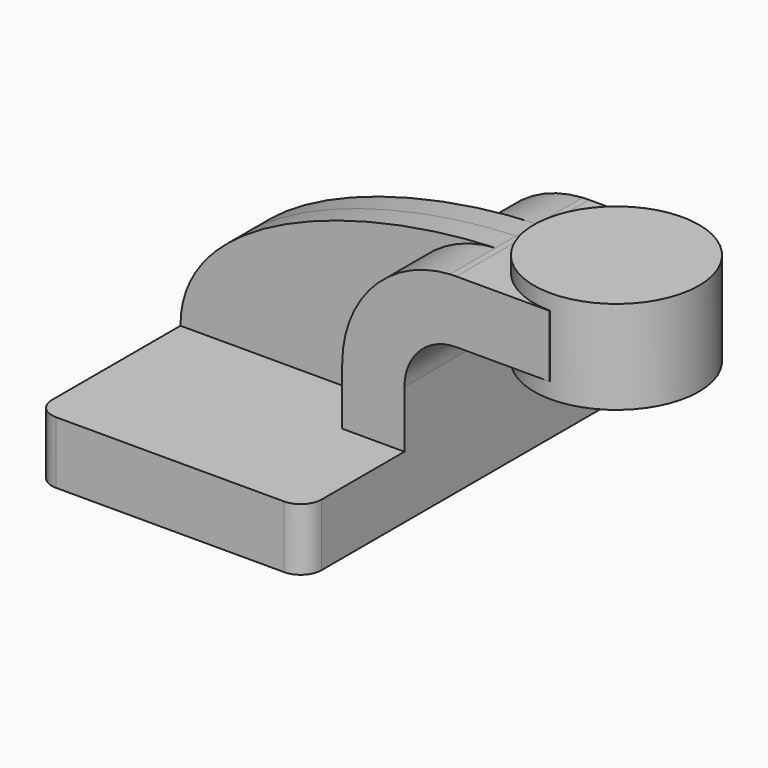
from build123d import *

# Parameters (mm, degrees)
F1_DEPTH = 63.5
F0_W     = 25.4
F0_H     = 19.05
F2_DEPTH = 25.4
F3_DEPTH = 7.9375
F6_R     = 6.35


with BuildPart() as f1:
    # F0 (on Front) → F1 (new body, symmetric)
    with BuildSketch(Plane.XZ):
        Polygon((-41.275, -9.525), (41.275, -9.525), (41.275, 9.525), (22.225, 9.525), (-41.275, 9.525), align=None)
    extrude(amount=F1_DEPTH, both=True)

    # F0 (on Front) → F2 (join, symmetric)
    with BuildSketch(Plane.XZ):
        with BuildLine():
            Line((22.225, 9.525), (41.275, 9.525))
            Line((41.275, 9.525), (41.275, 27.0002))
            ThreePointArc((41.275, 27.0002), (45.9246798487, 38.2255201513), (57.15, 42.8752))
            Line((57.15, 42.8752), (60.325, 42.8752))
            Line((60.325, 42.8752), (60.325, 61.9252))
            Line((60.325, 61.9252), (57.15, 61.9252))
            add(Edge.make_bspline(
                [(55.1794589503, 61.8695646769), (55.8399698658, 61.8922829135), (56.4969113909, 61.9108291292), (57.15, 61.9252)],
                knots=[109.7486555894, 109.7486555894, 109.7486555894, 109.7486555894, 111.5045361635, 111.5045361635, 111.5045361635, 111.5045361635], degree=3))
            ThreePointArc((55.1794589503, 61.8695646769), (31.7671635631, 50.9890982536), (22.225, 27.0002))
            Line((22.225, 27.0002), (22.225, 9.525))
        make_face()
        with Locations((73.025, 52.4002)):
            Rectangle(F0_W, F0_H)
    extrude(amount=F2_DEPTH, both=True)

    # F0 (on Front) → F3 (join, symmetric)
    with BuildSketch(Plane.XZ):
        with BuildLine():
            add(Edge.make_bspline(
                [(-41.275, 9.525), (-41.3334957388, 42.730852595), (13.8952246787, 60.4495957119), (55.1794589503, 61.8695646769)],
                knots=[0, 0, 0, 0, 109.7486555894, 109.7486555894, 109.7486555894, 109.7486555894], degree=3))
            Line((-41.275, 9.525), (22.225, 9.525))
            Line((22.225, 9.525), (22.225, 27.0002))
            ThreePointArc((22.225, 27.0002), (31.7671635631, 50.9890982536), (55.1794589503, 61.8695646769))
        make_face()
    extrude(amount=F3_DEPTH, both=True)

    # F6
    f6_edges = [f1.edges().sort_by_distance(p)[0] for p in [
        (41.275, 63.5, 0),
        (41.275, -63.5, 0),
        (-41.275, 63.5, 0),
        (-41.275, -63.5, 0),
    ]]
    fillet(f6_edges, radius=F6_R)


with BuildPart() as f5:
    # F4 (on face) → F5 (revolve)
    with BuildSketch(Plane.XZ):
        Polygon((85.8692377806, 66.675), (85.8692377806, 43.0761948228), (85.8692377806, 38.1), (111.125, 38.1), (111.125, 66.675), align=None)
    revolve(axis=Axis((85.8692377806, 0, 52.3519143462), (0, 0, -1)))


solid = Compound([f1.part, f5.part])
